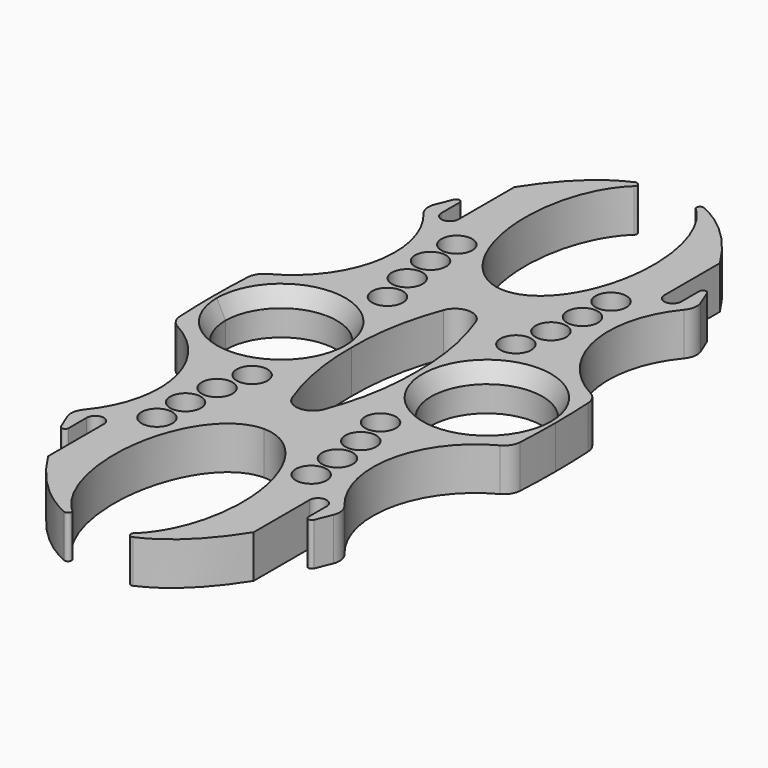
from build123d import *
from build123d import SkipClean  # not in build123d's __all__

# Parameters (mm, degrees)
F0_R        = 1.8
F1_DEPTH    = 5
F2_T1_DEPTH = 25.6143013412
F2_T3_DEPTH = 14.2800340441
F5_R        = 2
F6_SIZE2    = 1
F6_SIZE     = 2


# Not quite as in the source:
# - a fillet or chamfer that OpenCascade refuses, or shapes differently, is made with other operations: its cross-section is extruded or revolved along the edge and cut away or added
# - a feature names something its author has since deleted; it is built from what else it names


with BuildPart() as f1:
    # F0 (on Top) → F1 (new body)
    with BuildSketch(Plane.XY):
        with BuildLine():
            ThreePointArc((-5.5, 0), (-12, -6.5), (-18.5, 0))
            Line((-18.5, 0), (-20, 0))
            add(Edge.make_bspline(
                [(-20, 0), (-20, -3.0911979431), (-19.7895037833, -6.1498616127)],
                knots=[4.7123889804, 4.7123889804, 4.7123889804, 4.8576014094, 4.8576014094, 4.8576014094], degree=2, weights=[1, 0.9973653265, 1]))
            ThreePointArc((-19.7895037833, -6.1498616127), (-12.6830169424, -14.8586202596), (-15.9609156586, -25.6103648807))
            add(Edge.make_bspline(
                [(-15.9609156586, -25.6103648807), (-15.0629245494, -28.1375202449), (-13.9986054737, -30.3539752198)],
                knots=[5.3591400817, 5.3591400817, 5.3591400817, 5.5078854423, 5.5078854423, 5.5078854423], degree=2, weights=[1, 0.9972356268, 1]))
            Line((-13.9986054737, -30.3539752198), (-13.9986054737, -25.8696660557))
            ThreePointArc((-13.9986054737, -25.8696660557), (-12.9986054737, -24.8696660557), (-11.9986054737, -25.8696660557))
            Line((-11.9986054737, -25.8696660557), (-11.9986054737, -34.0022223246))
            add(Edge.make_bspline(
                [(-11.9986054737, -34.0022223246), (-6.6656982913, -42.5), (0, -42.5)],
                knots=[5.6397713534, 5.6397713534, 5.6397713534, 6.2831853072, 6.2831853072, 6.2831853072], degree=2, weights=[1, 0.9486970776, 1]))
            add(Edge.make_bspline(
                [(0, -17.5), (-7.5, -17.5), (-7.5, -30), (-7.5, -42.5), (0, -42.5)],
                knots=[3.1415926536, 3.1415926536, 3.1415926536, 4.7123889804, 4.7123889804, 6.2831853072, 6.2831853072, 6.2831853072], degree=2, weights=[1, 0.7071067812, 1, 0.7071067812, 1]))
            Line((0, -17.5), (0, -15.0755569339))
            ThreePointArc((0, -15.0755569339), (-2.8951406392, -7.7879867624), (-3.8104441483, 0))
            Line((-3.8104441483, 0), (-5.5, 0))
        make_face()
        with Locations((-8.9986054737, -21.8696660557)):
            Circle(F0_R, mode=Mode.SUBTRACT)
        with Locations((-8.864497038, -17.8696660557)):
            Circle(F0_R, mode=Mode.SUBTRACT)
        with Locations((-8.3848771, -13.8696660557)):
            Circle(F0_R, mode=Mode.SUBTRACT)
        with Locations((-7.4936952971, -9.8696660557)):
            Circle(F0_R, mode=Mode.SUBTRACT)
    extrude(amount=F1_DEPTH)

    # F2: fillet of radius 0.4 on 2 edges, made by hand

    # F2_s2 → F2_t1 (cut)
    with BuildSketch(Plane.XY.offset(-10.3071506706)):
        with BuildLine():
            ThreePointArc((-4.0297631159, -41.6288019622), (-3.5333540134, -41.4798515486), (-3.599456828, -40.965810071))
            Line((-3.599456828, -40.965810071), (-3.5724688033, -40.9362124681))
            ThreePointArc((-3.5724688033, -40.9362124681), (-1.9345357729, -42.0331443681), (0, -42.4599453926))
            Line((0, -42.4599453926), (0, -42.5400546074))
            ThreePointArc((0, -42.5400546074), (-2.069580304, -42.3128623444), (-4.04580572, -41.6655035484))
            Line((-4.04580572, -41.6655035484), (-4.0297631159, -41.6288019622))
        make_face()
    extrude(amount=F2_T1_DEPTH, mode=Mode.SUBTRACT)

    # F2_s4 → F2_t3 (cut)
    with BuildSketch(Plane.XY.offset(-4.6400170221)):
        with BuildLine():
            ThreePointArc((-14.7667367345, -28.6643789246), (-14.3179984189, -28.8985103868), (-13.9982054737, -28.5061889756))
            Line((-13.9982054737, -28.5061889756), (-13.9581508662, -28.5061889756))
            ThreePointArc((-13.9581508662, -28.5061889756), (-13.9585508662, -29.4300820977), (-13.9585508662, -30.3539752198))
            Line((-13.9585508662, -30.3539752198), (-14.0347129518, -30.3713136625))
            ThreePointArc((-14.0347129518, -30.3713136625), (-14.4277587718, -29.5296535334), (-14.8035352532, -28.6801979195))
            Line((-14.8035352532, -28.6801979195), (-14.7667367345, -28.6643789246))
        make_face()
    extrude(amount=F2_T3_DEPTH, mode=Mode.SUBTRACT)

    # F3: F1 across face


with BuildPart() as f1_1:
    add(f1.part, clean=False)
    add(f1.part.mirror(Plane(origin=(0, -16.2877784669, 2.5), x_dir=(0, 1, 0), z_dir=(1, 0, 0))), clean=False)

    # F4: F1 across face


with BuildPart() as f1_2:
    add(f1_1.part, clean=False)
    with SkipClean():  # cleaning this boolean's faces spoils the solid; the shape is the same uncleaned
        add(f1_1.part.mirror(Plane(origin=(-4.6552220741, 0, 2.5), x_dir=(-1, 0, 0), z_dir=(0, 1, 0))), clean=False)

    # F5
    f5_edges = [f1_2.edges().sort_by_distance(p)[0] for p in [
        (0, 15.075557, 2.5),
        (0, -15.075557, 2.5),
        (15.960916, -25.610365, 2.5),
        (15.960916, 25.610365, 2.5),
        (-15.960916, -25.610365, 2.5),
        (-15.960916, 25.610365, 2.5),
        (19.789504, -6.149862, 2.5),
        (19.789504, 6.149862, 2.5),
        (-19.789504, 6.149862, 2.5),
        (-19.789504, -6.149862, 2.5),
    ]]
    fillet(f5_edges, radius=F5_R)

    # F6
    f6_edges = [f1_2.edges().sort_by_distance(p)[0] for p in [
        (-12, -6.5, 5),
        (-12, 6.5, 5),
        (12, -6.5, 5),
        (12, 6.5, 5),
    ]]
    chamfer(f6_edges, length=F6_SIZE, length2=F6_SIZE2)


solid = f1_2.part
